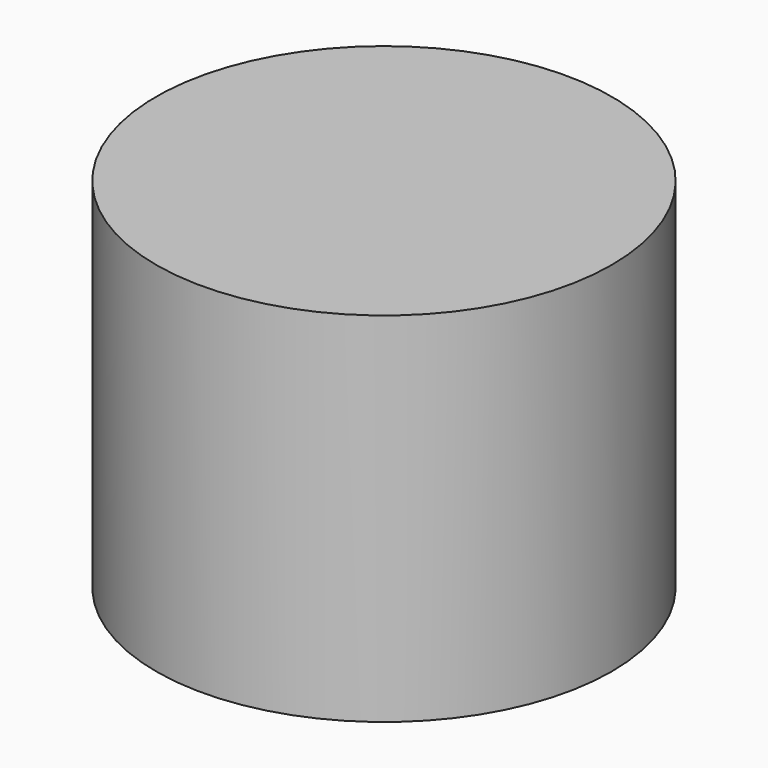
from build123d import *

# Parameters (mm, degrees)
F0_R     = 31.8248959205
F2_DEPTH = 50
F1_R     = 31.8248959205


# Not quite as in the source:
# - a feature of the source that left no trace in its solid (it failed there, or was rolled back) is left out


with BuildPart() as f2:
    # F0 (on Top) → F2 (new body)
    with BuildSketch(Plane.XY):
        Circle(F0_R)
    extrude(amount=F2_DEPTH)


with BuildPart() as f2b:
    # F1 (on face) → F2, piece 2 (new body)
    with BuildSketch(Plane.XY):
        Circle(F1_R)
    extrude(amount=F2_DEPTH)


solid = Compound([f2.part, f2b.part])
